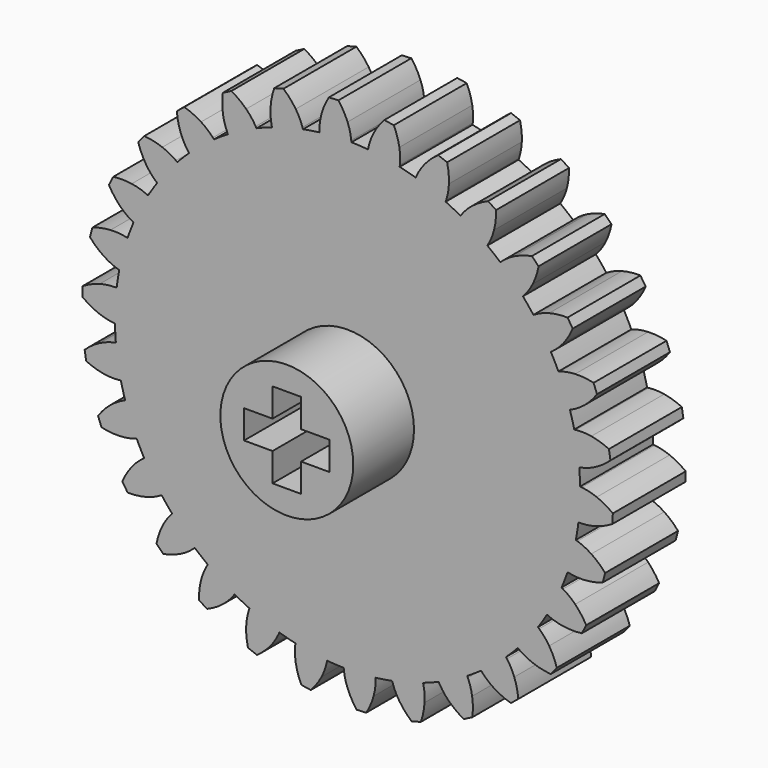
from build123d import *

# Parameters (mm, degrees)
F1_DEPTH = 9.6
F2_COUNT = 30
F3_R     = 10
F4_DEPTH = 5
F5_R     = 7
F6_DEPTH = 8
F5_W     = 3
F5_H     = 3
F7_DEPTH = 10


# Not quite as in the source:
# - a feature names something its author has since deleted; it is built from what else it names


with BuildPart() as f1:
    # F0 (on Front) → F1 (new body)
    with BuildSketch(Plane.XZ):
        with BuildLine():
            ThreePointArc((-2.9669573088, 24.3196867646), (-16.2412983769, -18.3431247892), (24.5, 0))
            ThreePointArc((24.5, 0), (17.467982293, 17.1790452182), (0.4086045216, 24.496592464))
            ThreePointArc((0.4086045216, 24.496592464), (-1.282230928, 24.4664236015), (-2.9669573088, 24.3196867646))
        make_face()
        with BuildLine():
            ThreePointArc((-2.9669573088, 24.3196867646), (-1.282230928, 24.4664236015), (0.4086045216, 24.496592464))
            ThreePointArc((0.4086045216, 24.496592464), (0.3967655337, 24.5818783933), (0.39065099, 24.6677647352))
            ThreePointArc((0.39065099, 24.6677647352), (0.2485851367, 25.4720320756), (0, 26.25))
            ThreePointArc((0, 26.25), (-0.4217786836, 27.1303085918), (-0.9599618272, 27.9446791333))
            Line((-0.9599618272, 27.9446791333), (-1.9663113104, 27.8919385917))
            ThreePointArc((-1.9663113104, 27.8919385917), (-2.4164213292, 27.0257738003), (-2.7438721608, 26.1061997534))
            ThreePointArc((-2.7438721608, 26.1061997534), (-2.9097757304, 25.3065093964), (-2.966994503, 24.4917979913))
            ThreePointArc((-2.966994503, 24.4917979913), (-2.9640979832, 24.4057429999), (-2.9669573088, 24.3196867646))
        make_face()
    extrude(amount=F1_DEPTH)


with BuildPart() as f2_1:
    # F2: instance of F1
    add(f1.part.rotate(Axis((0, 0, 0), (0, -1, 0)), 1 * 360 / F2_COUNT))


with BuildPart() as f2_2:
    # F2: instance of F1
    add(f1.part.rotate(Axis((0, 0, 0), (0, -1, 0)), 2 * 360 / F2_COUNT))


with BuildPart() as f2_3:
    # F2: instance of F1
    add(f1.part.rotate(Axis((0, 0, 0), (0, -1, 0)), 3 * 360 / F2_COUNT))


with BuildPart() as f2_4:
    # F2: instance of F1
    add(f1.part.rotate(Axis((0, 0, 0), (0, -1, 0)), 4 * 360 / F2_COUNT))


with BuildPart() as f2_5:
    # F2: instance of F1
    add(f1.part.rotate(Axis((0, 0, 0), (0, -1, 0)), 5 * 360 / F2_COUNT))


with BuildPart() as f2_6:
    # F2: instance of F1
    add(f1.part.rotate(Axis((0, 0, 0), (0, -1, 0)), 6 * 360 / F2_COUNT))


with BuildPart() as f2_7:
    # F2: instance of F1
    add(f1.part.rotate(Axis((0, 0, 0), (0, -1, 0)), 7 * 360 / F2_COUNT))


with BuildPart() as f2_8:
    # F2: instance of F1
    add(f1.part.rotate(Axis((0, 0, 0), (0, -1, 0)), 8 * 360 / F2_COUNT))


with BuildPart() as f2_9:
    # F2: instance of F1
    add(f1.part.rotate(Axis((0, 0, 0), (0, -1, 0)), 9 * 360 / F2_COUNT))


with BuildPart() as f2_10:
    # F2: instance of F1
    add(f1.part.rotate(Axis((0, 0, 0), (0, -1, 0)), 10 * 360 / F2_COUNT))


with BuildPart() as f2_11:
    # F2: instance of F1
    add(f1.part.rotate(Axis((0, 0, 0), (0, -1, 0)), 11 * 360 / F2_COUNT))


with BuildPart() as f2_12:
    # F2: instance of F1
    add(f1.part.rotate(Axis((0, 0, 0), (0, -1, 0)), 12 * 360 / F2_COUNT))


with BuildPart() as f2_13:
    # F2: instance of F1
    add(f1.part.rotate(Axis((0, 0, 0), (0, -1, 0)), 13 * 360 / F2_COUNT))


with BuildPart() as f2_14:
    # F2: instance of F1
    add(f1.part.rotate(Axis((0, 0, 0), (0, -1, 0)), 14 * 360 / F2_COUNT))


with BuildPart() as f2_15:
    # F2: instance of F1
    add(f1.part.rotate(Axis((0, 0, 0), (0, -1, 0)), 15 * 360 / F2_COUNT))


with BuildPart() as f2_16:
    # F2: instance of F1
    add(f1.part.rotate(Axis((0, 0, 0), (0, -1, 0)), 16 * 360 / F2_COUNT))


with BuildPart() as f2_17:
    # F2: instance of F1
    add(f1.part.rotate(Axis((0, 0, 0), (0, -1, 0)), 17 * 360 / F2_COUNT))


with BuildPart() as f2_18:
    # F2: instance of F1
    add(f1.part.rotate(Axis((0, 0, 0), (0, -1, 0)), 18 * 360 / F2_COUNT))


with BuildPart() as f2_19:
    # F2: instance of F1
    add(f1.part.rotate(Axis((0, 0, 0), (0, -1, 0)), 19 * 360 / F2_COUNT))


with BuildPart() as f2_20:
    # F2: instance of F1
    add(f1.part.rotate(Axis((0, 0, 0), (0, -1, 0)), 20 * 360 / F2_COUNT))


with BuildPart() as f2_21:
    # F2: instance of F1
    add(f1.part.rotate(Axis((0, 0, 0), (0, -1, 0)), 21 * 360 / F2_COUNT))


with BuildPart() as f2_22:
    # F2: instance of F1
    add(f1.part.rotate(Axis((0, 0, 0), (0, -1, 0)), 22 * 360 / F2_COUNT))


with BuildPart() as f2_23:
    # F2: instance of F1
    add(f1.part.rotate(Axis((0, 0, 0), (0, -1, 0)), 23 * 360 / F2_COUNT))


with BuildPart() as f2_24:
    # F2: instance of F1
    add(f1.part.rotate(Axis((0, 0, 0), (0, -1, 0)), 24 * 360 / F2_COUNT))


with BuildPart() as f2_25:
    # F2: instance of F1
    add(f1.part.rotate(Axis((0, 0, 0), (0, -1, 0)), 25 * 360 / F2_COUNT))


with BuildPart() as f2_26:
    # F2: instance of F1
    add(f1.part.rotate(Axis((0, 0, 0), (0, -1, 0)), 26 * 360 / F2_COUNT))


with BuildPart() as f2_27:
    # F2: instance of F1
    add(f1.part.rotate(Axis((0, 0, 0), (0, -1, 0)), 27 * 360 / F2_COUNT))


with BuildPart() as f2_28:
    # F2: instance of F1
    add(f1.part.rotate(Axis((0, 0, 0), (0, -1, 0)), 28 * 360 / F2_COUNT))


with BuildPart() as f2_29:
    # F2: instance of F1
    add(f1.part.rotate(Axis((0, 0, 0), (0, -1, 0)), 29 * 360 / F2_COUNT))


with BuildPart() as f1_1:
    add(f1.part)

    add(f2_1.part)  # F4 merges F2_1

    add(f2_2.part)  # F4 merges F2_2

    add(f2_3.part)  # F4 merges F2_3

    add(f2_4.part)  # F4 merges F2_4

    add(f2_5.part)  # F4 merges F2_5

    add(f2_6.part)  # F4 merges F2_6

    add(f2_7.part)  # F4 merges F2_7

    add(f2_8.part)  # F4 merges F2_8

    add(f2_9.part)  # F4 merges F2_9

    add(f2_10.part)  # F4 merges F2_10

    add(f2_11.part)  # F4 merges F2_11

    add(f2_12.part)  # F4 merges F2_12

    add(f2_13.part)  # F4 merges F2_13

    add(f2_14.part)  # F4 merges F2_14

    add(f2_15.part)  # F4 merges F2_15

    add(f2_16.part)  # F4 merges F2_16

    add(f2_17.part)  # F4 merges F2_17

    add(f2_18.part)  # F4 merges F2_18

    add(f2_19.part)  # F4 merges F2_19

    add(f2_20.part)  # F4 merges F2_20

    add(f2_21.part)  # F4 merges F2_21

    add(f2_22.part)  # F4 merges F2_22

    add(f2_23.part)  # F4 merges F2_23

    add(f2_24.part)  # F4 merges F2_24

    add(f2_25.part)  # F4 merges F2_25

    add(f2_26.part)  # F4 merges F2_26

    add(f2_27.part)  # F4 merges F2_27

    add(f2_28.part)  # F4 merges F2_28

    add(f2_29.part)  # F4 merges F2_29
    # F3 (on face) → F4 (join)
    with BuildSketch(Plane(origin=(0, 0, 0), x_dir=(-1, 0, 0), z_dir=(0, 1, 0))):
        Circle(F3_R)
    extrude(amount=F4_DEPTH)

    # F5 (on face) → F6 (join)
    with BuildSketch(Plane.XZ.offset(9.6)):
        Circle(F5_R)
        Polygon((-4.5, -1.5), (-4.5, 1.5), (-1.5, 1.5), (-1.5, 4.5), (1.5, 4.5), (1.5, 1.5), (4.5, 1.5), (4.5, -1.5), (1.5, -1.5), (1.5, -4.5), (-1.5, -4.5), (-1.5, -1.5), align=None, mode=Mode.SUBTRACT)
    extrude(amount=F6_DEPTH)

    # F5 (on face) → F7 (cut)
    with BuildSketch(Plane.XZ.offset(9.6)):
        with Locations((-3, 0)):
            Rectangle(F5_W, F5_H)
        with Locations((0, 3)):
            Rectangle(F5_W, F5_H)
        with Locations((3, 0)):
            Rectangle(F5_W, F5_H)
        Rectangle(F5_W, F5_H)
        with Locations((0, -3)):
            Rectangle(F5_W, F5_H)
    extrude(amount=-F7_DEPTH, mode=Mode.SUBTRACT)


solid = f1_1.part
